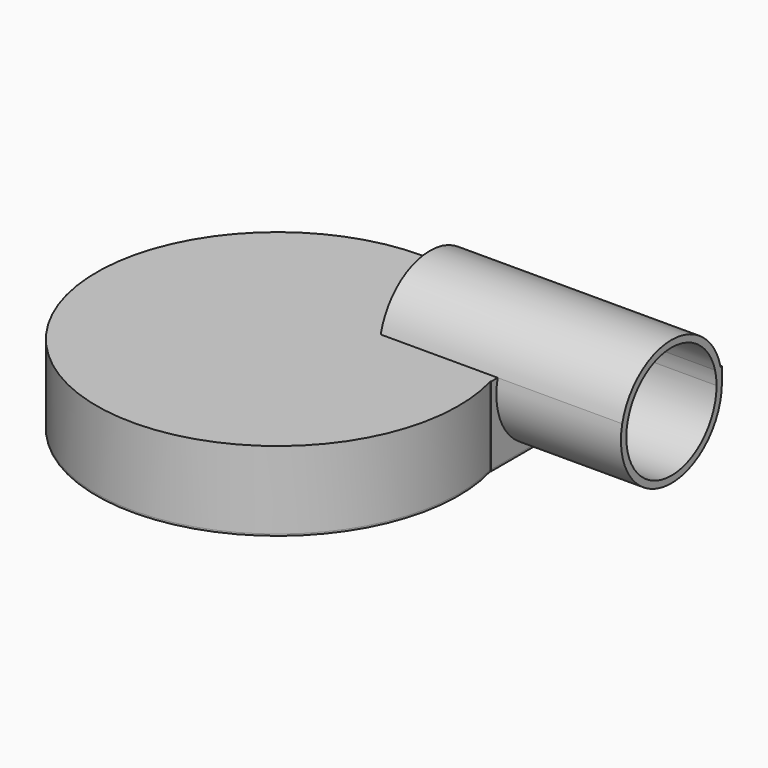
from build123d import *
from build123d import SkipClean  # not in build123d's __all__

# Parameters (mm, degrees)
F1_DEPTH = 46
F3_DEPTH = 74
F4_DEPTH = 143.5
F5_R     = 75
F5_R_2   = 72
F6_DEPTH = 40
F7_R     = 72
F8_DEPTH = 1


# Not quite as in the source:
# - after a boolean that leaves OpenCascade's solid faulty, fix() repairs it


with BuildPart() as f1:
    # F0 (on Top) → F1 (new body)
    with BuildSketch(Plane.XY):
        with BuildLine():
            Line((178, 107.5), (0, 107.5))
            ThreePointArc((0, 107.5), (-65.1632565178, -85.4985379992), (103.6532681588, 28.5))
            Line((103.6532681588, 28.5), (178, 28.5))
            Line((178, 28.5), (178, 107.5))
        make_face()
    extrude(amount=F1_DEPTH)

    # F2 (on face) → F3 (cut)
    with BuildSketch(Plane.YZ.offset(178)):
        with BuildLine():
            ThreePointArc((70, 0), (40.6316496888, 14.1815523673), (33.4760352645, 46))
            Line((33.4760352645, 46), (28.5, 46))
            Line((28.5, 46), (28.5, 0))
            Line((28.5, 0), (70, 0))
        make_face()
        with BuildLine():
            Line((107.5, 0), (107.5, 37.5))
            ThreePointArc((107.5, 37.5), (96.5165042945, 10.9834957055), (70, 0))
            Line((70, 0), (107.5, 0))
        make_face()
        with BuildLine():
            ThreePointArc((37.596296508, 46), (65.714796795, 4.275204538), (103.5, 37.5))
            ThreePointArc((103.5, 37.5), (103.224795462, 41.785203205), (102.403703492, 46))
            Line((102.403703492, 46), (37.596296508, 46))
        make_face()
    extrude(amount=-F3_DEPTH, mode=Mode.SUBTRACT)

    # F2 (on face) → F4 (join)
    with BuildSketch(Plane.YZ.offset(178)):
        with BuildLine():
            ThreePointArc((37.596296508, 46), (70, 71), (102.403703492, 46))
            Line((102.403703492, 46), (106.5239647355, 46))
            ThreePointArc((106.5239647355, 46), (70, 75), (33.4760352645, 46))
            Line((33.4760352645, 46), (37.596296508, 46))
        make_face()
    with SkipClean():  # cleaning this boolean's faces spoils the solid; the shape is the same uncleaned
        extrude(amount=-F4_DEPTH)

    # F5 (on face) → F6 (cut)
    with BuildSketch(Plane(origin=(0, 0, 0), x_dir=(1, 0, 0), z_dir=(0, 0, -1))):
        with BuildLine():
            ThreePointArc((98.8321859189, -27.1744186047), (-62.1324073774, 81.5218618132), (0, -102.5))
            Line((0, -102.5), (98.8321859189, -102.5))
            Line((98.8321859189, -102.5), (98.8321859189, -27.1744186047))
        make_face()
        Circle(F5_R, mode=Mode.SUBTRACT)
        Circle(F5_R_2)
    extrude(amount=-F6_DEPTH, mode=Mode.SUBTRACT)

    add(f1.part.fix(), mode=Mode.REPLACE)

    # F7 (on face) → F8 (join)
    with BuildSketch(Plane(origin=(0, 0, 0), x_dir=(1, 0, 0), z_dir=(0, 0, -1))):
        with BuildLine():
            ThreePointArc((103.6532681588, -28.5), (-65.1632565178, 85.4985379992), (0, -107.5))
            Line((0, -107.5), (104, -107.5))
            Line((104, -107.5), (104, -70))
            Line((104, -70), (104, -28.5))
            Line((104, -28.5), (103.6532681588, -28.5))
        make_face()
        with BuildLine():
            ThreePointArc((0, -102.5), (-62.1324073774, 81.5218618132), (98.8321859189, -27.1744186047))
            Line((98.8321859189, -27.1744186047), (98.8321859189, -102.5))
            Line((98.8321859189, -102.5), (0, -102.5))
        make_face(mode=Mode.SUBTRACT)
        with BuildLine():
            Line((98.8321859189, -102.5), (98.8321859189, -27.1744186047))
            ThreePointArc((98.8321859189, -27.1744186047), (-62.1324073774, 81.5218618132), (0, -102.5))
            Line((0, -102.5), (98.8321859189, -102.5))
        make_face()
        Circle(F7_R, mode=Mode.SUBTRACT)
    extrude(amount=F8_DEPTH)


solid = f1.part
